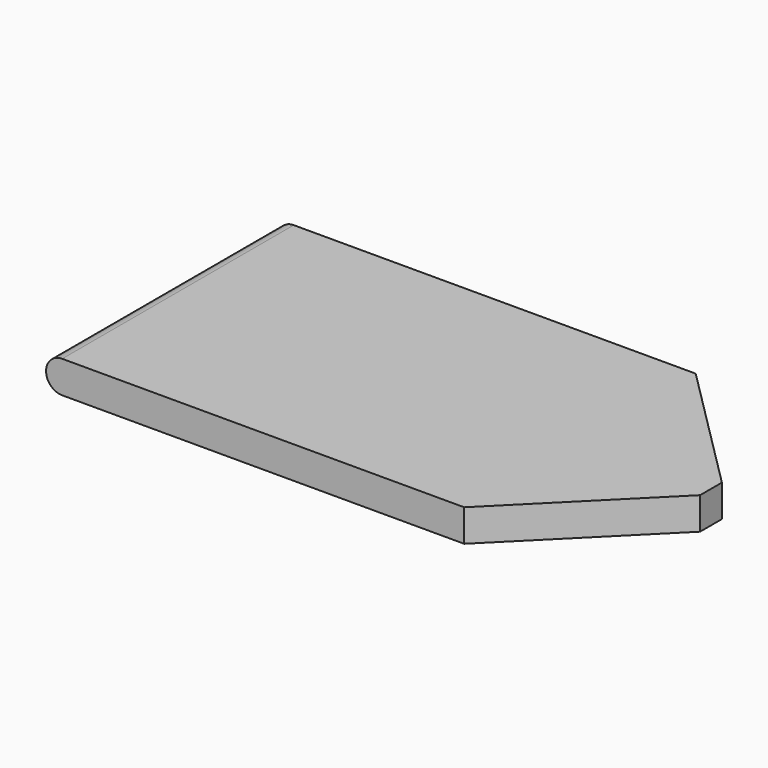
from build123d import *

# Parameters (mm, degrees)
F1_DEPTH    = 12.7
F2_D        = 5.08
F2_DEPTH    = 5.08
F2_TIP      = 1.5261859723
F3_D        = 5.08
F3_DEPTH    = 5.08
F3_TIP      = 1.5261859723
F4_T1_DEPTH = 339.3037394717
F5_SIZE     = 7.62
F6_R        = 6.34999


# Not quite as in the source:
# - a fillet or chamfer that OpenCascade refuses, or shapes differently, is made with other operations: its cross-section is extruded or revolved along the edge and cut away or added
# - a fillet or chamfer is up to 0.001 mm smaller than in the source, because OpenCascade refuses the exact size


with BuildPart() as f1:
    # F0 (on Top) → F1 (new body)
    with BuildSketch(Plane.XY):
        Polygon((114.3, 27.94), (114.3, 57.15), (82.55, 57.15), (-114.3, 57.15), (-114.3, -57.15), (82.55, -57.15), (114.3, -57.15), (114.3, -27.94), align=None)
    extrude(amount=F1_DEPTH)

    # F2
    with Locations(Plane(origin=(0, 0, 0), x_dir=(1, 0, 0), z_dir=(0, 0, -1))):
        with Locations((-65.25006, 0)):
            Hole(F2_D / 2, depth=F2_DEPTH)
            with Locations((0, 0, -(F2_DEPTH + F2_TIP / 2))):  # 118° drill point
                Cone(0, F2_D / 2, F2_TIP, mode=Mode.SUBTRACT)

    # F3
    with Locations(Plane(origin=(0, 0, 0), x_dir=(1, 0, 0), z_dir=(0, 0, -1))):
        with Locations((0, 0), (65.25006, 0)):
            Hole(F3_D / 2, depth=F3_DEPTH)
            with Locations((0, 0, -(F3_DEPTH + F3_TIP / 2))):  # 118° drill point
                Cone(0, F3_D / 2, F3_TIP, mode=Mode.SUBTRACT)

    # F4: chamfer of 63.5 on 2 edges, made by hand

    # F4_s2 → F4_t1 (cut)
    with BuildSketch(Plane.XY.offset(-163.3018697358)):
        Polygon((114.3, -6.35), (50.8, 57.15), (114.3, 57.15), align=None)
        Polygon((114.3, 6.35), (50.8, -57.15), (114.3, -57.15), align=None)
    extrude(amount=F4_T1_DEPTH, mode=Mode.SUBTRACT)

    # F5
    f5_edges = [f1.edges().sort_by_distance(p)[0] for p in [
        (107.95, 0, 6.35),
    ]]
    chamfer(f5_edges, length=F5_SIZE)

    # F6 (radius 6.35 in the source; OpenCascade refuses exactly that, so slightly less here)
    f6_edges = [f1.edges().sort_by_distance(p)[0] for p in [
        (-114.3, 0, 0),
        (-114.3, 0, 12.7),
    ]]
    fillet(f6_edges, radius=F6_R)


solid = f1.part
